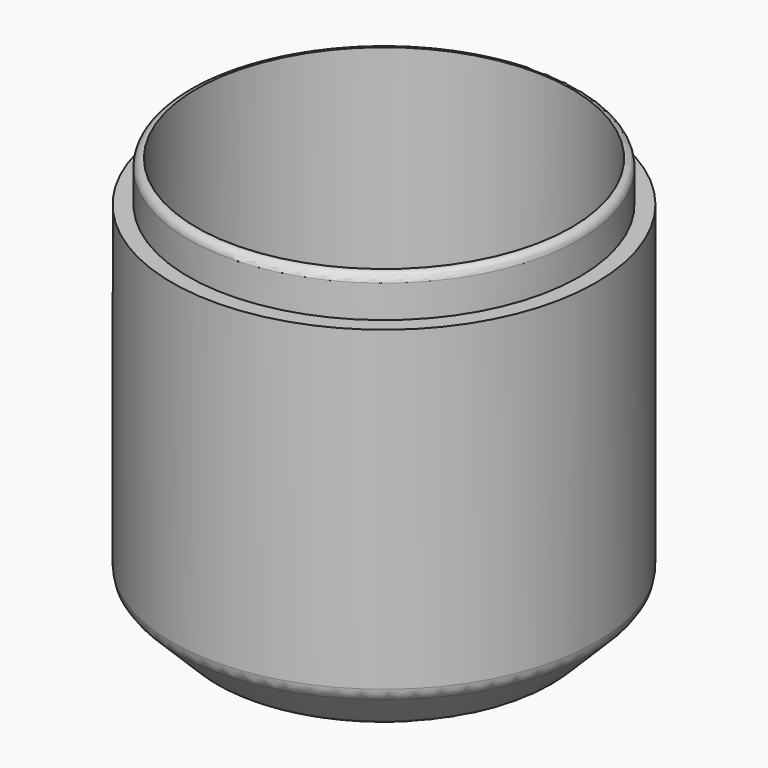
from build123d import *

# Parameters (mm, degrees)
F0_R     = 33.04
F1_DEPTH = 58
F2_SIZE  = 7.62
F3_T     = -3.81
F4_R     = 2.54
F5_R     = 30.5
F5_R_2   = 29.23
F6_DEPTH = 6.35
F7_R     = 1.26999


# Not quite as in the source:
# - a fillet or chamfer is up to 0.001 mm smaller than in the source, because OpenCascade refuses the exact size


with BuildPart() as f1:
    # F0 (on Top) → F1 (new body)
    with BuildSketch(Plane.XY):
        Circle(F0_R)
    extrude(amount=F1_DEPTH)

    # F2
    f2_edges = [f1.edges().sort_by_distance(p)[0] for p in [
        (-33.04, 0, 0),
    ]]
    chamfer(f2_edges, length=F2_SIZE)

    # F3
    f3_openings = [f1.faces().sort_by_distance(p)[0] for p in [
        (0, 0, 58),
    ]]
    offset(amount=F3_T, openings=f3_openings)

    # F4
    f4_edges = [f1.edges().sort_by_distance(p)[0] for p in [
        (-33.04, 0, 7.62),
        (-25.42, 0, 0),
    ]]
    fillet(f4_edges, radius=F4_R)

    # F5 (on face) → F6 (join)
    with BuildSketch(Plane.XY.offset(58)):
        Circle(F5_R)
        Circle(F5_R_2, mode=Mode.SUBTRACT)
    extrude(amount=F6_DEPTH)

    # F7 (radius 1.27 in the source; OpenCascade refuses exactly that, so slightly less here)
    f7_edges = [f1.edges().sort_by_distance(p)[0] for p in [
        (-30.5, 0, 64.35),
    ]]
    fillet(f7_edges, radius=F7_R)


solid = f1.part
